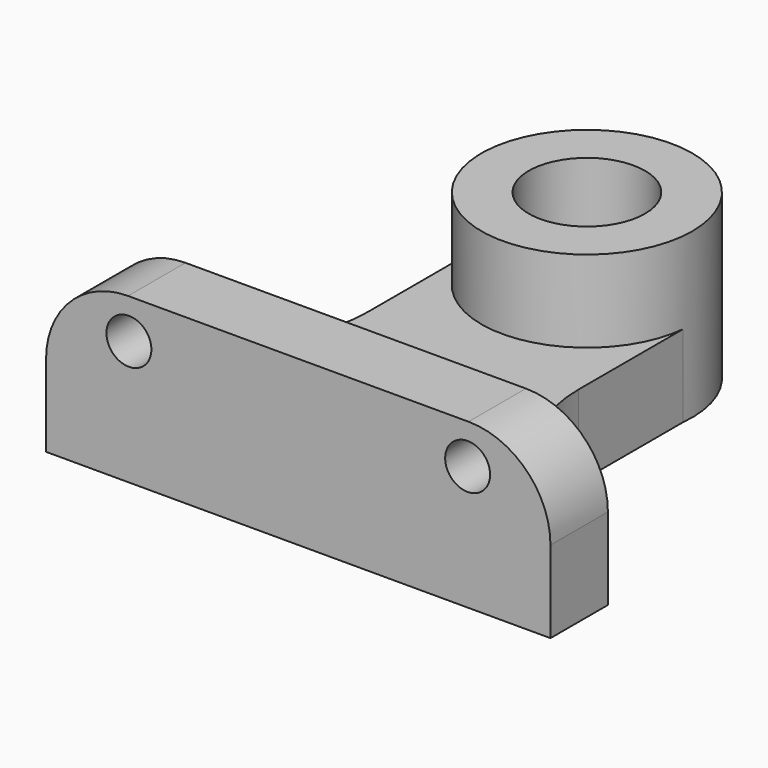
from build123d import *

# Parameters (mm, degrees)
F0_W     = 78.1559348106
F0_H     = 11.1243845895
F1_DEPTH = 25.4
F0_R     = 9.006561322
F2_DEPTH = 12.7
F3_R     = 12.7
F4_R     = 3.4818048238
F5_DEPTH = 11.1253845895


# Not quite as in the source:
# - ends of sketch curves that miss each other by under 0.0002 mm in the source are joined


with BuildPart() as f1:
    # F0 (on Top) → F1 (new body)
    with BuildSketch(Plane.XY):
        Rectangle(F0_W, F0_H)
    extrude(amount=F1_DEPTH)



with BuildPart() as f1b:
    # F0 (on Top) → F1, piece 2 (new body)
    with BuildSketch(Plane.XY):
        with BuildLine():
            Line((-16.3389042508, 50.9063668795), (-16.3389042508, 49.7835881762))
            ThreePointArc((-16.3389042508, 49.7835881762), (-0.5764210141, 34.0065966737), (16.2587184459, 48.6335381866))
            ThreePointArc((16.2587184459, 48.6335381866), (1.1371213689, 66.6539292144), (-16.3389042508, 50.9063668795))
        make_face()
        with Locations((0, 50.3449775279)):
            Circle(F0_R, mode=Mode.SUBTRACT)
    extrude(amount=F1_DEPTH)


with BuildPart() as f1_1:
    add(f1.part)

    add(f1b.part)  # F2 merges F1b
    # F0 (on Top) → F2 (join)
    with BuildSketch(Plane.XY):
        with BuildLine():
            ThreePointArc((-16.3389042508, 28.4221922947), (-23.0344432329, 12.2577312768), (-39.1989042508, 5.5621922947))
            Line((-39.1989042508, 5.5621922947), (-39.0779674053, 5.5621922947))
            Line((-39.0779674053, 5.5621922947), (39.0779674053, 5.5621922947))
            ThreePointArc((39.0779674053, 5.5621922947), (22.9398561975, 12.2721453491), (16.2587184459, 28.4221922947))
            Line((16.2587184459, 28.4221922947), (16.2587184459, 48.6335381866))
            ThreePointArc((16.2587184459, 48.6335381866), (-0.5764210141, 34.0065966737), (-16.3389042508, 49.7835881762))
            Line((-16.3389042508, 49.7835881762), (-16.3389042508, 28.4221922947))
        make_face()
    extrude(amount=F2_DEPTH)

    # F3
    f3_edges = [f1_1.edges().sort_by_distance(p)[0] for p in [
        (39.077967, 0, 25.4),
        (-39.077967, 0, 25.4),
    ]]
    fillet(f3_edges, radius=F3_R)

    # F4 (on face) → F5 (cut, through all)
    with BuildSketch(Plane(origin=(0, 5.5621922947, 0), x_dir=(-1, 0, 0), z_dir=(0, 1, 0))):
        with Locations((-26.2421388179, 19.2537438124)):
            Circle(F4_R)
        with Locations((26.2421388179, 19.2537438124)):
            Circle(F4_R)
    extrude(amount=-F5_DEPTH, mode=Mode.SUBTRACT)


solid = f1_1.part
